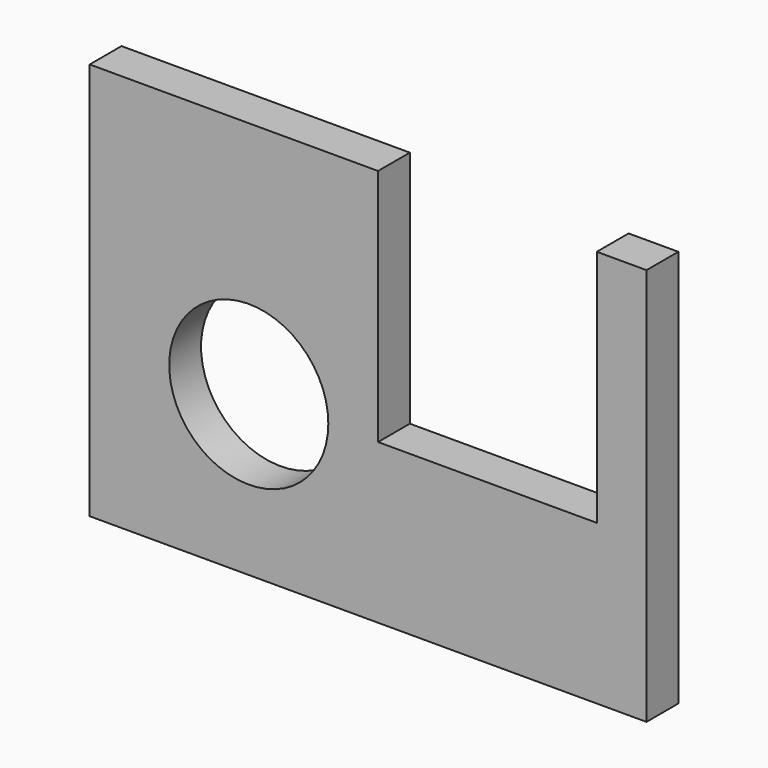
from build123d import *

# Parameters (mm, degrees)
F0_R     = 25.4
F1_DEPTH = 12.7


# Not quite as in the source:
# - a length typed as a fraction of an inch, garbled in the dataset ("3 / 203.2 mm" for 3/8 in), is restored


with BuildPart() as f1:
    # F0 (on Front) → F1 (new body)
    with BuildSketch(Plane.XZ):
        Polygon((-3.9472851508, 53.245825498), (-96.0222851508, 53.245825498), (-96.0222851508, -73.754174502), (81.7777148492, -73.754174502), (81.7777148492, 53.245825498), (65.9027148492, 53.245825498), (65.9027148492, -22.954174502), (-3.9472851508, -22.954174502), align=None)
        with Locations((-45.2222851508, -22.954174502)):
            Circle(F0_R, mode=Mode.SUBTRACT)
    extrude(amount=F1_DEPTH)


solid = f1.part
